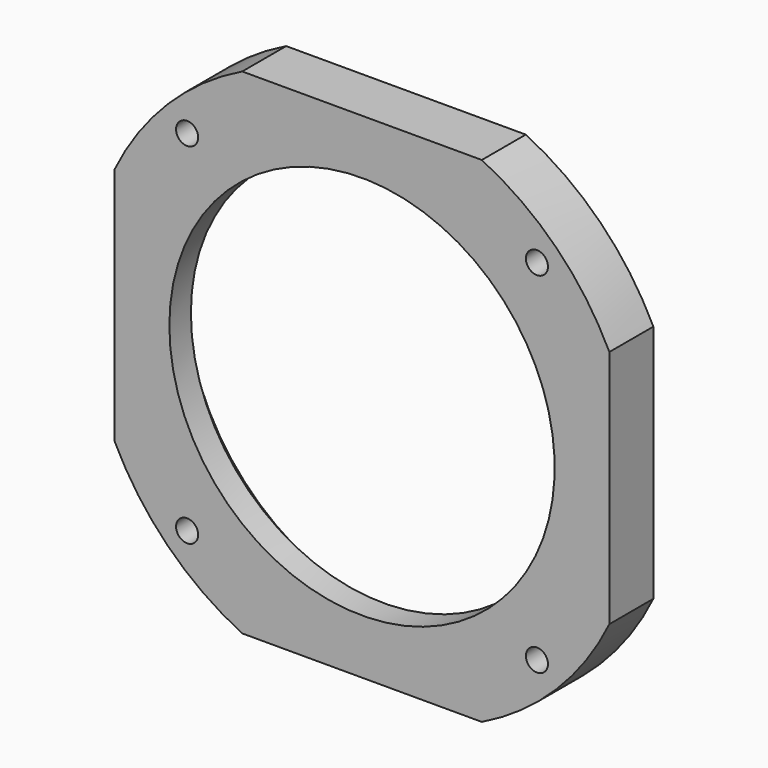
from build123d import *

# Parameters (mm, degrees)
F0_W      = 114.3
F0_H      = 114.3
F1_DEPTH  = 12.7
F2_R      = 50.8635
F3_DEPTH  = 6.477
F4_R      = 44.5135
F5_DEPTH  = 6.224
F6_R      = 9.525
F8_D      = 5.1054
F9_R      = 110.5427806282
F9_R_2    = 63.5
F10_DEPTH = 25.4
F12_D     = 5.1054


with BuildPart() as f1:
    # F0 (on Front) → F1 (new body)
    with BuildSketch(Plane.XZ):
        Rectangle(F0_W, F0_H)
    extrude(amount=-F1_DEPTH)

    # F2 (on face) → F3 (cut)
    with BuildSketch(Plane(origin=(0, 12.7, 0), x_dir=(-1, 0, 0), z_dir=(0, 1, 0))):
        Circle(F2_R)
    extrude(amount=-F3_DEPTH, mode=Mode.SUBTRACT)

    # F4 (on face) → F5 (cut, through all)
    with BuildSketch(Plane(origin=(0, 6.223, 0), x_dir=(-1, 0, 0), z_dir=(0, 1, 0))):
        Circle(F4_R)
    extrude(amount=-F5_DEPTH, mode=Mode.SUBTRACT)

    # F6
    f6_edges = [f1.edges().sort_by_distance(p)[0] for p in [
        (57.15, 6.35, 57.15),
        (-57.15, 6.35, 57.15),
        (57.15, 6.35, -57.15),
        (-57.15, 6.35, -57.15),
    ]]
    fillet(f6_edges, radius=F6_R)

    # F8 (through all)
    with Locations(Plane(origin=(0, 12.7, 0), x_dir=(-1, 0, 0), z_dir=(0, 1, 0))):
        with Locations((-47.625, 47.625), (47.625, -47.625), (47.625, 47.625), (-47.625, -47.625)):
            Hole(F8_D / 2)

    # F9 (on Front) → F10 (cut)
    with BuildSketch(Plane.XZ):
        Circle(F9_R)
        Circle(F9_R_2, mode=Mode.SUBTRACT)
    extrude(amount=-F10_DEPTH, mode=Mode.SUBTRACT)

    # F12 (through all)
    with Locations(Plane(origin=(0, 12.7, 0), x_dir=(-1, 0, 0), z_dir=(0, 1, 0))):
        with Locations((40.4111525448, 40.4111525448), (-40.4111525448, 40.4111525448), (-40.4111525448, -40.4111525448), (40.4111525448, -40.4111525448)):
            Hole(F12_D / 2)


solid = f1.part
